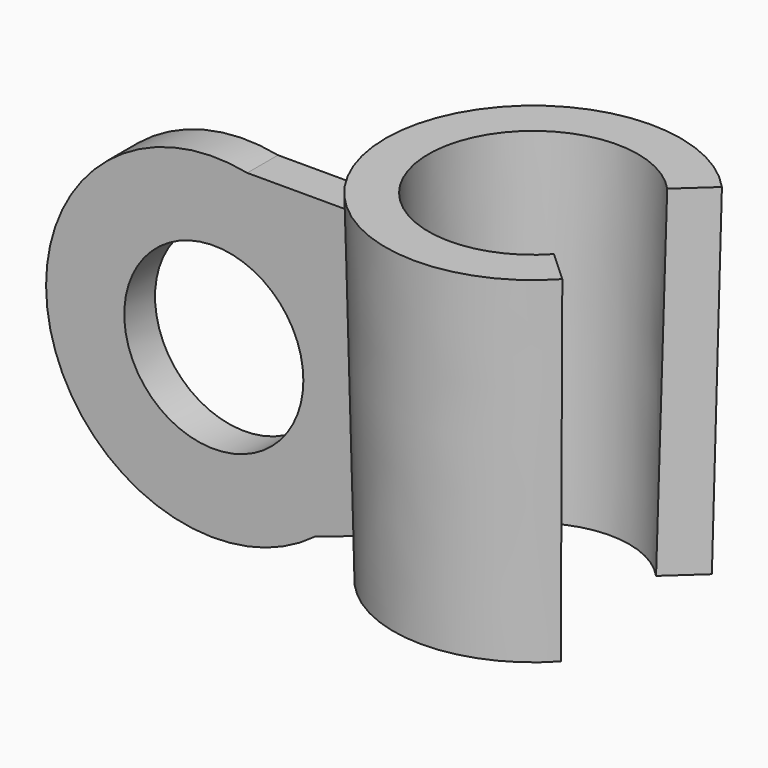
from build123d import *

# Parameters (mm, degrees)
F2_ANGLE_BACK = 137.5
F2_ANGLE      = 275
F3_R          = 10.25
F4_DEPTH      = 2.2
F5_T1_DEPTH   = 4.4


# Not quite as in the source:
# - a fillet or chamfer that OpenCascade refuses, or shapes differently, is made with other operations: its cross-section is extruded or revolved along the edge and cut away or added


with BuildPart() as f2:
    # F1 (on Front) → F2 (revolve)
    with BuildSketch(Plane.XZ, mode=Mode.PRIVATE) as f2_sk:
        Polygon((-11, 0), (-12, 38.9871773792), (-16.9010080012, 38.9871773792), (-16, 0), align=None)
    revolve(f2_sk.sketch.rotate(Axis((0, 0, 0), (0, 0, 1)), -F2_ANGLE_BACK), axis=Axis((0, 0, 0), (0, 0, 1)), revolution_arc=F2_ANGLE)

    # F3 (on Front) → F4 (join, symmetric)
    with BuildSketch(Plane.XZ):
        with BuildLine():
            ThreePointArc((-20.6759724746, 0), (-16.9178855504, 6.0230564645), (-15.6053744435, 13))
            ThreePointArc((-15.6053744435, 13), (-19.938561129, 25.149809129), (-30.9822350551, 31.8155150133))
            ThreePointArc((-30.9822350551, 31.8155150133), (-53.0709208133, 7.0830906875), (-20.6759724746, 0))
        make_face()
        with Locations((-34.8053744435, 13)):
            Circle(F3_R, mode=Mode.SUBTRACT)
        with BuildLine():
            ThreePointArc((-30.9822350551, 31.8155150133), (-19.938561129, 25.149809129), (-15.6053744435, 13))
            ThreePointArc((-15.6053744435, 13), (-16.9178855504, 6.0230564645), (-20.6759724746, 0))
            Line((-20.6759724746, 0), (-15.4107194394, 0))
            Line((-15.4107194394, 0), (-15.4107194394, 31.8155150133))
            Line((-15.4107194394, 31.8155150133), (-30.9822350551, 31.8155150133))
        make_face()
    extrude(amount=F4_DEPTH, both=True)

    # F5: chamfer of 5 on 1 edges, made by hand

    # F5_s2 → F5_t1 (join)
    with BuildSketch(Plane.XZ.offset(-2.2)):
        with BuildLine():
            Line((-16.1513787733, 0.0636631161), (-23.407451394, -2.3727904591))
            Line((-23.407451394, -2.3727904591), (-23.4678030607, -2.2930554208))
            ThreePointArc((-23.4678030607, -2.2930554208), (-22.0304116691, -1.1989551063), (-20.7495631098, 0.0677083333))
            Line((-20.7495631098, 0.0677083333), (-20.6759724746, 0.1))
            ThreePointArc((-20.6759724746, 0.1), (-18.413675624, 0.1), (-16.1513787733, 0.1636631161))
            Line((-16.1513787733, 0.1636631161), (-16.1513787733, 0.0636631161))
        make_face()
    extrude(amount=F5_T1_DEPTH)


solid = f2.part
